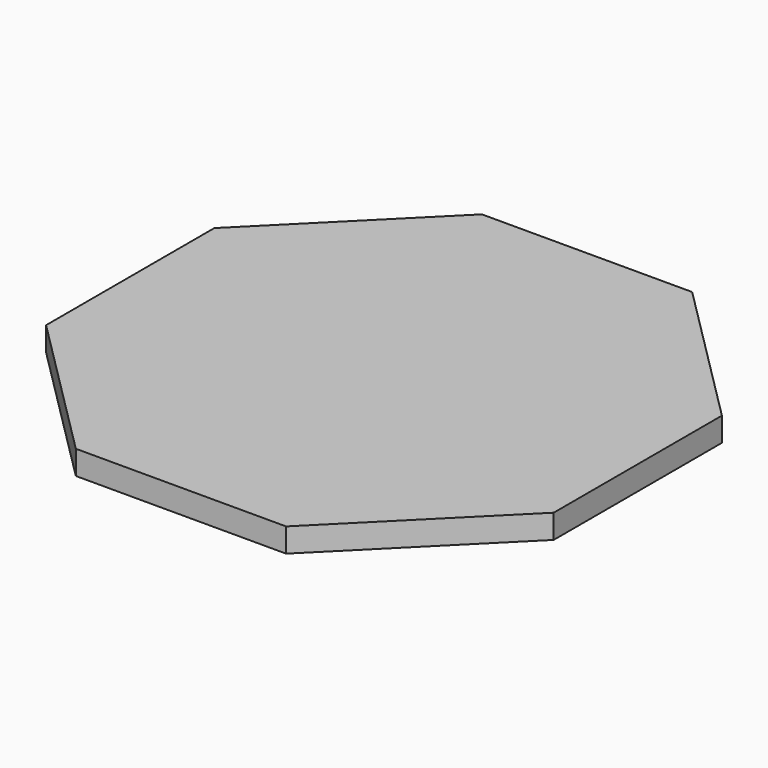
from build123d import *

# Parameters (mm, degrees)
F1_DEPTH = 19.05


# Not quite as in the source:
# - a feature names something its author has since deleted; it is built from what else it names


with BuildPart() as f1:
    # F0 (on Top) → F1 (new body)
    with BuildSketch(Plane.XY):
        Polygon((-83.5106318439, -201.6125), (83.5106318439, -201.6125), (201.6125, -83.5106318439), (201.6125, 83.5106318439), (83.5106318439, 201.6125), (-83.5106318439, 201.6125), (-201.6125, 83.5106318439), (-201.6125, -83.5106318439), align=None)
    extrude(amount=F1_DEPTH)


solid = f1.part
